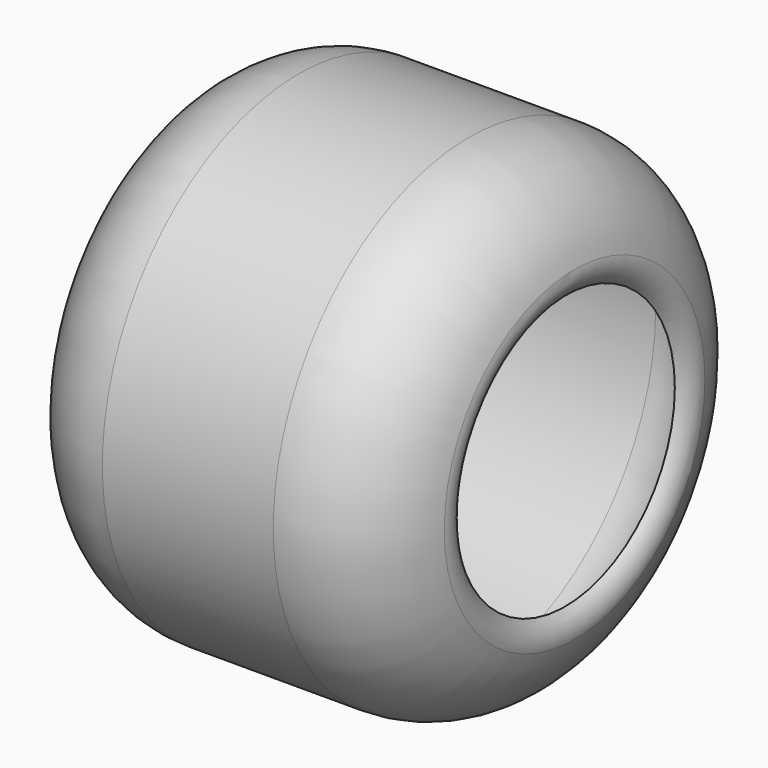
from build123d import *

# Parameters (mm, degrees)
F0_R     = 50
F1_DEPTH = 78.994
F2_R     = 22.0755688143
F3_T     = -2.54


# Not quite as in the source:
# - a fillet or chamfer that OpenCascade refuses, or shapes differently, is made with other operations: its cross-section is extruded or revolved along the edge and cut away or added


with BuildPart() as f1:
    # F0 (on Right) → F1 (new body)
    with BuildSketch(Plane.YZ):
        Circle(F0_R)
    extrude(amount=F1_DEPTH)

    # F2
    f2_edges = [f1.edges().sort_by_distance(p)[0] for p in [
        (78.994, -50, 0),
        (0, -50, 0),
        (39.497, 50, 0),
    ]]
    fillet(f2_edges, radius=F2_R)

    # F3: a shell. OpenCascade refuses it in one call, so the cavity is built on its own and cut out:
    # the body offset inwards by the wall thickness, plus a prism from it out through each open face.
    f3_core = offset(f1.part, amount=F3_T, mode=Mode.PRIVATE)
    f3_exits = [f3_core.faces().sort_by_distance(p)[0] for p in [
        (76.454, 0, 0),
        (2.54, 0, 0),
    ]]
    add(f3_core, mode=Mode.SUBTRACT)
    extrude(f3_exits, amount=-F3_T, mode=Mode.SUBTRACT)

    # F4: fillet of radius 5.08 on 6 edges, made by hand

    # F4_s1 → F4_t2 (revolve, cut)
    with BuildSketch(Plane.XY):
        with BuildLine():
            ThreePointArc((0.6434411467, 33.2154275111), (0.793307898, 30.2837381407), (2.54, 27.9244311857))
            Line((2.54, 27.9244311857), (0, 27.9244311857))
            ThreePointArc((0, 27.9244311857), (0.1614506751, 30.5894198641), (0.6434411467, 33.2154275111))
        make_face()
    revolve(axis=Axis((0, 0, 0), (1, 0, 0)), mode=Mode.SUBTRACT)

    # F4_s3 → F4_t4 (revolve, cut)
    with BuildSketch(Plane.XY):
        with BuildLine():
            ThreePointArc((78.3505588533, 33.2154275111), (78.200692102, 30.2837381407), (76.454, 27.9244311857))
            Line((76.454, 27.9244311857), (78.994, 27.9244311857))
            ThreePointArc((78.994, 27.9244311857), (78.8325493249, 30.5894198641), (78.3505588533, 33.2154275111))
        make_face()
    revolve(axis=Axis((78.994, 0, 0), (1, 0, 0)), mode=Mode.SUBTRACT)


solid = f1.part
